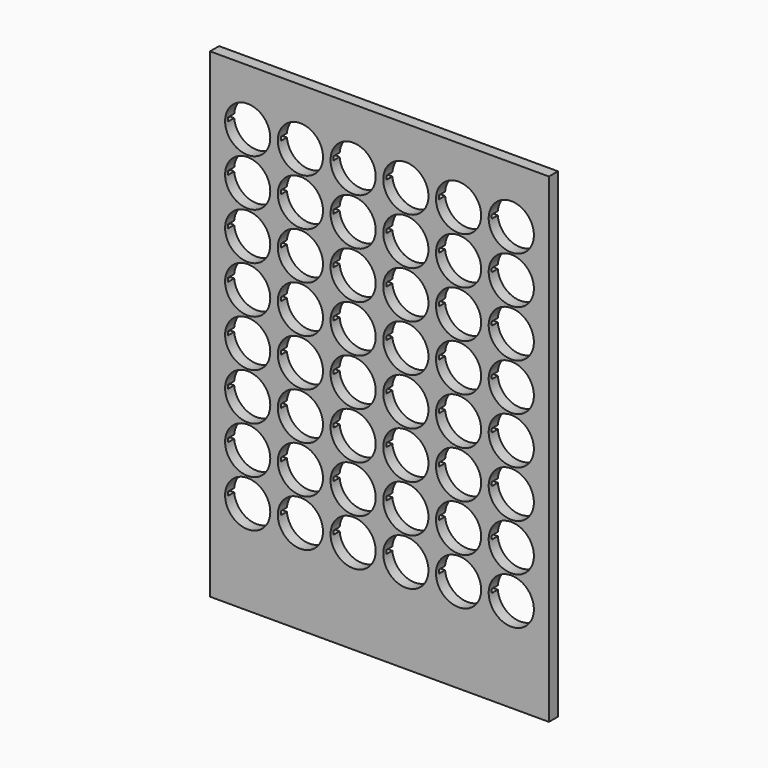
from build123d import *

# Parameters (mm, degrees)
F0_W     = 180
F0_H     = 255
F0_R     = 12
F1_DEPTH = 6
F3_W     = 168
F3_H     = 2
F4_DEPTH = 4


# Not quite as in the source:
# - a feature names something its author has since deleted; it is built from what else it names


with BuildPart() as f1:
    # F0 (on Front) → F1 (new body)
    with BuildSketch(Plane.XZ):
        Rectangle(F0_W, F0_H)
        with Locations((-70, -77.5)):
            Circle(F0_R, mode=Mode.SUBTRACT)
        with Locations((-42, -77.5)):
            Circle(F0_R, mode=Mode.SUBTRACT)
        with Locations((-14, -77.5)):
            Circle(F0_R, mode=Mode.SUBTRACT)
        with Locations((-70, -52.5)):
            Circle(F0_R, mode=Mode.SUBTRACT)
        with Locations((-70, -27.5)):
            Circle(F0_R, mode=Mode.SUBTRACT)
        with Locations((-70, -2.5)):
            Circle(F0_R, mode=Mode.SUBTRACT)
        with Locations((-42, -52.5)):
            Circle(F0_R, mode=Mode.SUBTRACT)
        with Locations((-14, -52.5)):
            Circle(F0_R, mode=Mode.SUBTRACT)
        with Locations((-42, -27.5)):
            Circle(F0_R, mode=Mode.SUBTRACT)
        with Locations((-42, -2.5)):
            Circle(F0_R, mode=Mode.SUBTRACT)
        with Locations((-14, -27.5)):
            Circle(F0_R, mode=Mode.SUBTRACT)
        with Locations((-14, -2.5)):
            Circle(F0_R, mode=Mode.SUBTRACT)
        with Locations((14, -77.5)):
            Circle(F0_R, mode=Mode.SUBTRACT)
        with Locations((42, -77.5)):
            Circle(F0_R, mode=Mode.SUBTRACT)
        with Locations((70, -77.5)):
            Circle(F0_R, mode=Mode.SUBTRACT)
        with Locations((14, -52.5)):
            Circle(F0_R, mode=Mode.SUBTRACT)
        with Locations((42, -52.5)):
            Circle(F0_R, mode=Mode.SUBTRACT)
        with Locations((14, -27.5)):
            Circle(F0_R, mode=Mode.SUBTRACT)
        with Locations((14, -2.5)):
            Circle(F0_R, mode=Mode.SUBTRACT)
        with Locations((42, -27.5)):
            Circle(F0_R, mode=Mode.SUBTRACT)
        with Locations((42, -2.5)):
            Circle(F0_R, mode=Mode.SUBTRACT)
        with Locations((70, -52.5)):
            Circle(F0_R, mode=Mode.SUBTRACT)
        with Locations((70, -27.5)):
            Circle(F0_R, mode=Mode.SUBTRACT)
        with Locations((70, -2.5)):
            Circle(F0_R, mode=Mode.SUBTRACT)
        with Locations((-70, 22.5)):
            Circle(F0_R, mode=Mode.SUBTRACT)
        with Locations((-70, 47.5)):
            Circle(F0_R, mode=Mode.SUBTRACT)
        with Locations((-42, 22.5)):
            Circle(F0_R, mode=Mode.SUBTRACT)
        with Locations((-14, 22.5)):
            Circle(F0_R, mode=Mode.SUBTRACT)
        with Locations((-42, 47.5)):
            Circle(F0_R, mode=Mode.SUBTRACT)
        with Locations((-14, 47.5)):
            Circle(F0_R, mode=Mode.SUBTRACT)
        with Locations((-70, 72.5)):
            Circle(F0_R, mode=Mode.SUBTRACT)
        with Locations((-70, 97.5)):
            Circle(F0_R, mode=Mode.SUBTRACT)
        with Locations((-42, 72.5)):
            Circle(F0_R, mode=Mode.SUBTRACT)
        with Locations((-14, 72.5)):
            Circle(F0_R, mode=Mode.SUBTRACT)
        with Locations((-42, 97.5)):
            Circle(F0_R, mode=Mode.SUBTRACT)
        with Locations((-14, 97.5)):
            Circle(F0_R, mode=Mode.SUBTRACT)
        with Locations((14, 22.5)):
            Circle(F0_R, mode=Mode.SUBTRACT)
        with Locations((42, 22.5)):
            Circle(F0_R, mode=Mode.SUBTRACT)
        with Locations((14, 47.5)):
            Circle(F0_R, mode=Mode.SUBTRACT)
        with Locations((42, 47.5)):
            Circle(F0_R, mode=Mode.SUBTRACT)
        with Locations((70, 22.5)):
            Circle(F0_R, mode=Mode.SUBTRACT)
        with Locations((70, 47.5)):
            Circle(F0_R, mode=Mode.SUBTRACT)
        with Locations((14, 72.5)):
            Circle(F0_R, mode=Mode.SUBTRACT)
        with Locations((42, 72.5)):
            Circle(F0_R, mode=Mode.SUBTRACT)
        with Locations((14, 97.5)):
            Circle(F0_R, mode=Mode.SUBTRACT)
        with Locations((42, 97.5)):
            Circle(F0_R, mode=Mode.SUBTRACT)
        with Locations((70, 72.5)):
            Circle(F0_R, mode=Mode.SUBTRACT)
        with Locations((70, 97.5)):
            Circle(F0_R, mode=Mode.SUBTRACT)
    extrude(amount=F1_DEPTH)

    # F3 (on face) → F4 (cut)
    with BuildSketch(Plane.XZ):
        with Locations((0, 97.5)):
            Rectangle(F3_W, F3_H)
        with Locations((0, 72.5)):
            Rectangle(F3_W, F3_H)
        with Locations((0, 47.5)):
            Rectangle(F3_W, F3_H)
        with Locations((0, 22.5)):
            Rectangle(F3_W, F3_H)
        with Locations((0, -2.5)):
            Rectangle(F3_W, F3_H)
        with Locations((0, -27.5)):
            Rectangle(F3_W, F3_H)
        with Locations((0, -52.5)):
            Rectangle(F3_W, F3_H)
        with Locations((0, -77.5)):
            Rectangle(F3_W, F3_H)
    extrude(amount=F4_DEPTH, mode=Mode.SUBTRACT)


solid = f1.part
